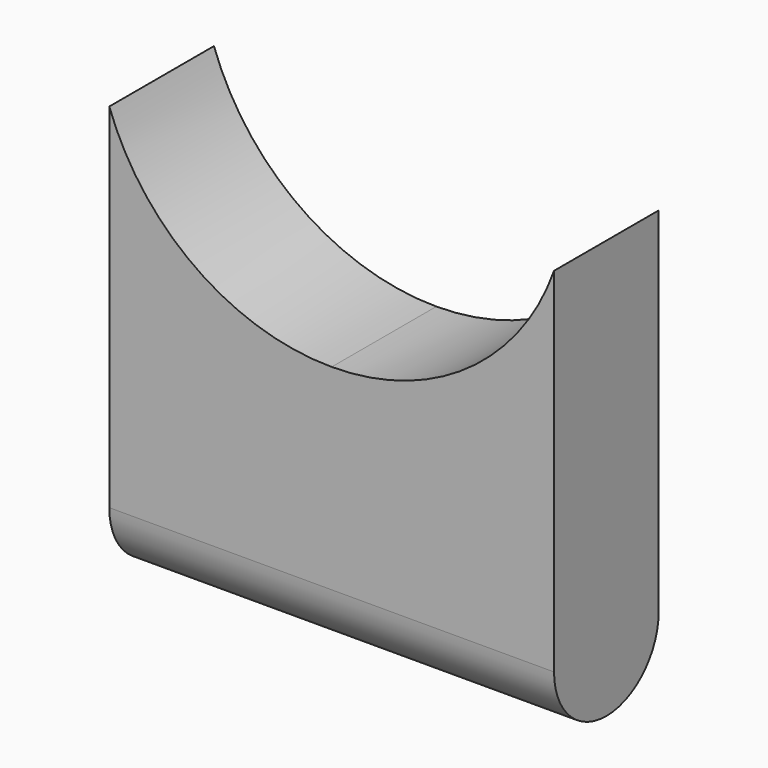
from build123d import *

# Parameters (mm, degrees)
F1_DEPTH = 10
F2_R     = 4.99999


# Not quite as in the source:
# - a fillet or chamfer is up to 0.001 mm smaller than in the source, because OpenCascade refuses the exact size


with BuildPart() as f1:
    # F0 (on Front) → F1 (new body)
    with BuildSketch(Plane.XZ):
        with BuildLine():
            Line((34, -32), (34, 0))
            ThreePointArc((34, 0), (27.4043260233, -8.6977951997), (17, -12))
            ThreePointArc((17, -12), (6.5956739767, -8.6977951997), (0, 0))
            Line((0, 0), (0, -5))
            Line((0, -5), (0, -32))
            Line((0, -32), (34, -32))
        make_face()
    extrude(amount=F1_DEPTH)

    # F2 (radius 5 in the source; OpenCascade refuses exactly that, so slightly less here)
    f2_edges = [f1.edges().sort_by_distance(p)[0] for p in [
        (17, 0, -32),
        (17, -10, -32),
    ]]
    fillet(f2_edges, radius=F2_R)


solid = f1.part
